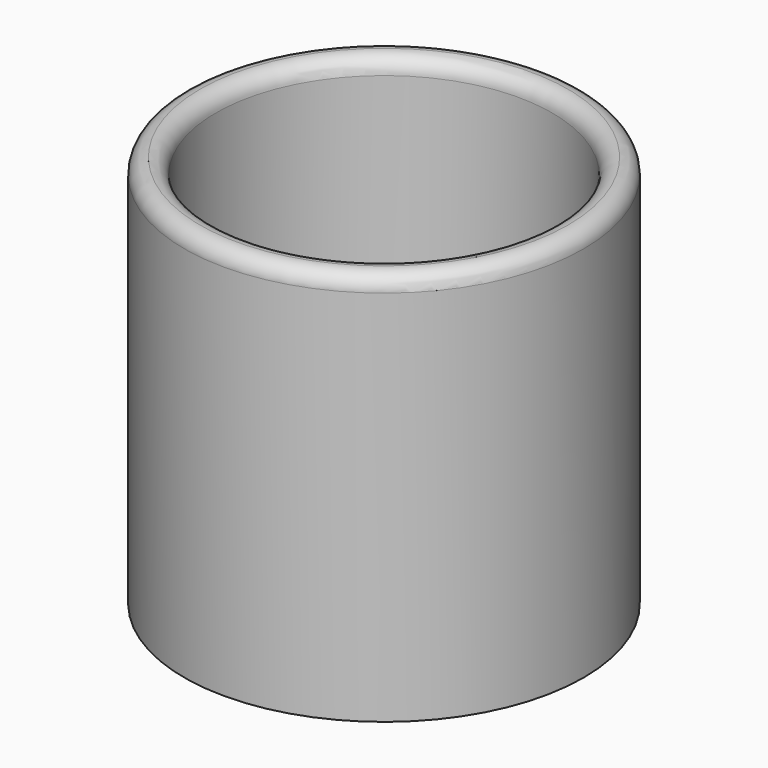
from build123d import *

# Parameters (mm, degrees)
F0_R     = 25.4
F0_R_2   = 21.4
F1_DEPTH = 50
F2_R     = 1.99999


# Not quite as in the source:
# - a fillet or chamfer is up to 0.001 mm smaller than in the source, because OpenCascade refuses the exact size


with BuildPart() as f1:
    # F0 (on Top) → F1 (new body)
    with BuildSketch(Plane.XY):
        Circle(F0_R)
        Circle(F0_R_2, mode=Mode.SUBTRACT)
    extrude(amount=F1_DEPTH)

    # F2 (radius 2 in the source; OpenCascade refuses exactly that, so slightly less here)
    f2_edges = [f1.edges().sort_by_distance(p)[0] for p in [
        (-25.4, 0, 50),
        (-21.4, 0, 50),
    ]]
    fillet(f2_edges, radius=F2_R)


solid = f1.part
